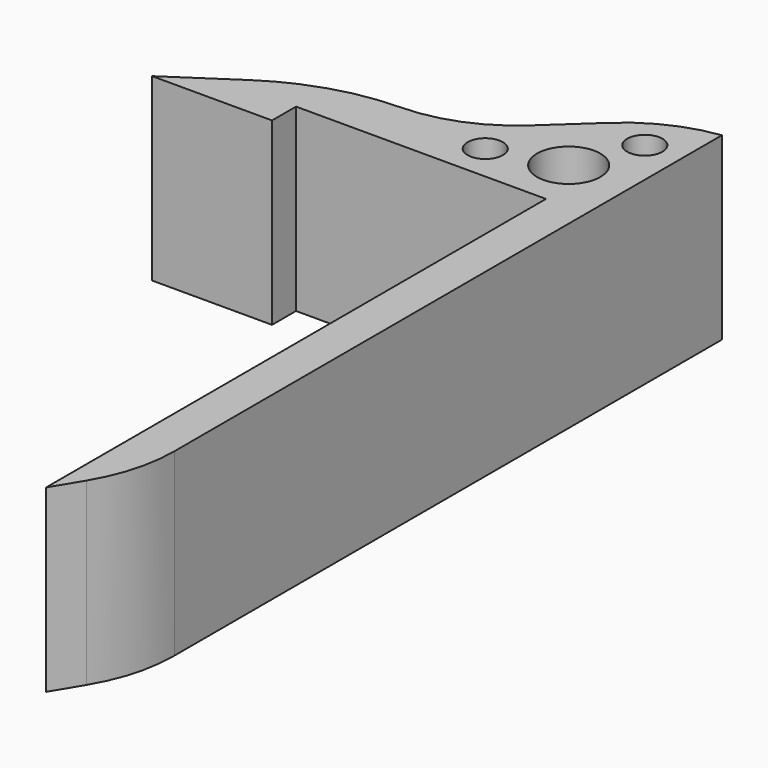
from build123d import *

# Parameters (mm, degrees)
F1_DEPTH    = 18
F2_T1_DEPTH = 18
F2_T3_DEPTH = 46.2017417965
F3_R        = 22.3056916506
F4_R        = 15.8040911287
F5_R        = 1.7635852265
F5_R_2      = 3.1709752344
F6_DEPTH    = 18


# Not quite as in the source:
# - a fillet or chamfer that OpenCascade refuses, or shapes differently, is made with other operations: its cross-section is extruded or revolved along the edge and cut away or added


with BuildPart() as f1:
    # F0 (on Top) → F1 (new body)
    with BuildSketch(Plane.XY):
        Polygon((-17.5491029148, 7.6061424899), (7.4508970852, 7.6061424899), (7.4508970852, -54.8938575101), (11.4508970852, -48.259973526), (11.4508970852, 24.6061424899), (7.4508970852, 24.6061424899), (-5.5491029148, 12.6061424899), (-17.5491029148, 12.6061424899), (-29.5491029148, 4.6061424899), (-17.5491029148, 4.6061424899), align=None)
    extrude(amount=F1_DEPTH)

    # F2: fillet of radius 14.9219158343 on 2 edges, made by hand

    # F2_s2 → F2_t1 (join)
    with BuildSketch(Plane.XY):
        with BuildLine():
            ThreePointArc((-11.3833307845, 12.6061424899), (-5.9496574254, 13.6306209347), (-1.2620921794, 16.5633831687))
            Line((-1.2620921794, 16.5633831687), (-5.5491029148, 12.6061424899))
            Line((-5.5491029148, 12.6061424899), (-11.3833307845, 12.6061424899))
        make_face()
    extrude(amount=F2_T1_DEPTH)

    # F2_s4 → F2_t3 (cut)
    with BuildSketch(Plane.XY.offset(-14.1008708982)):
        with BuildLine():
            ThreePointArc((11.4508970852, 24.6061424899), (7.0833751355, 23.32182366), (3.3063496819, 20.7804064253))
            Line((3.3063496819, 20.7804064253), (7.4508970852, 24.6061424899))
            Line((7.4508970852, 24.6061424899), (11.4508970852, 24.6061424899))
        make_face()
    extrude(amount=F2_T3_DEPTH, mode=Mode.SUBTRACT)

    # F3
    f3_edges = [f1.edges().sort_by_distance(p)[0] for p in [
        (-17.549103, 12.606142, 9),
    ]]
    fillet(f3_edges, radius=F3_R)

    # F4
    f4_edges = [f1.edges().sort_by_distance(p)[0] for p in [
        (11.450897, -48.259974, 9),
    ]]
    fillet(f4_edges, radius=F4_R)

    # F5 (on face) → F6 (cut)
    with BuildSketch(Plane.XY.offset(18)):
        with Locations((-1.5691251028, 11.2882275134)):
            Circle(F5_R)
        with Locations((5.2787014283, 13.1632275879)):
            Circle(F5_R_2)
        with Locations((7.8058750369, 19.5219237357)):
            Circle(F5_R)
    extrude(amount=-F6_DEPTH, mode=Mode.SUBTRACT)


solid = f1.part
